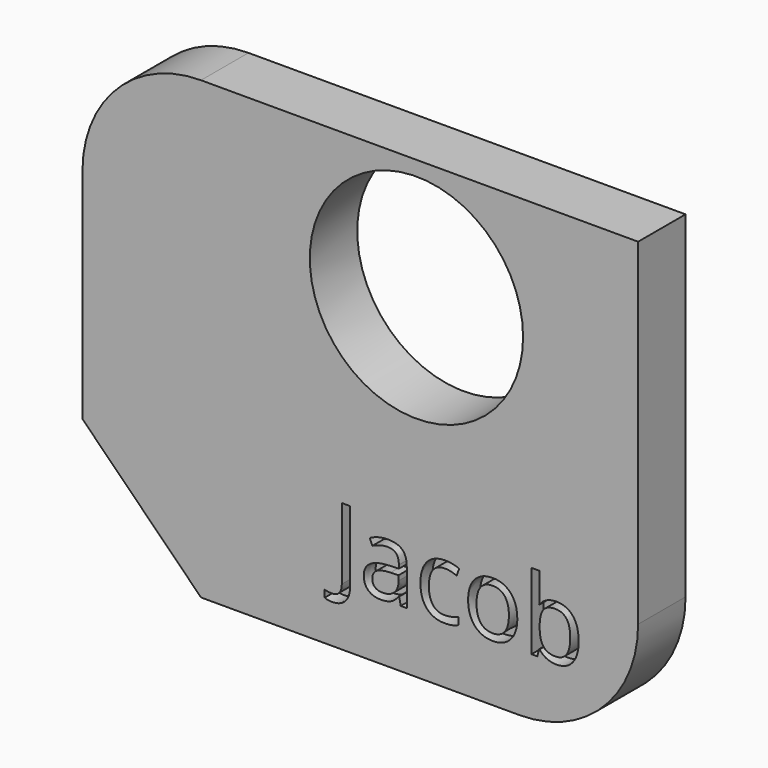
from build123d import *

# Parameters (mm, degrees)
F0_W         = 95.2185168862
F0_H         = 78.0262835324
F1_DEPTH     = 10.16
F2_R         = 18.272587144
F3_DEPTH     = 25.4
F4_R         = 20.32
F5_R         = 20.32
F6_SIZE      = 20.32
F7_TEXT_SIZE = 17.1441222645
F8_DEPTH     = 2.54


# Not quite as in the source:
# - Text() gives the source's letters only with a copy of the font that has no kerning and outlines rounded to 1/6400 em; it was checked with that copy


with BuildPart() as f1:
    # F0 (on Front) → F1 (new body)
    with BuildSketch(Plane.XZ):
        with Locations((2.5127120316, -6.7446436733)):
            Rectangle(F0_W, F0_H)
    extrude(amount=F1_DEPTH)

    # F2 (on face) → F3 (cut)
    with BuildSketch(Plane.XZ.offset(10.16)):
        with Locations((12.1352532879, 11.4783784375)):
            Circle(F2_R)
    extrude(amount=-F3_DEPTH, mode=Mode.SUBTRACT)

    # F4
    f4_edges = [f1.edges().sort_by_distance(p)[0] for p in [
        (-45.096546, -5.08, 32.268498),
    ]]
    fillet(f4_edges, radius=F4_R)

    # F5
    f5_edges = [f1.edges().sort_by_distance(p)[0] for p in [
        (50.12197, -5.08, -45.757785),
    ]]
    fillet(f5_edges, radius=F5_R)

    # F6
    f6_edges = [f1.edges().sort_by_distance(p)[0] for p in [
        (-45.096546, -5.08, -45.757785),
    ]]
    chamfer(f6_edges, length=F6_SIZE)

    # F7 (on face) → F8 (cut)
    with BuildSketch(Plane.XZ.offset(10.16)):
        with Locations((-2.2482152563, -35.9002351761)):
            Text('Jacob', F7_TEXT_SIZE, font='Open Sans', text_align=(TextAlign.LEFT, TextAlign.BOTTOM))
    extrude(amount=-F8_DEPTH, mode=Mode.SUBTRACT)


solid = f1.part
